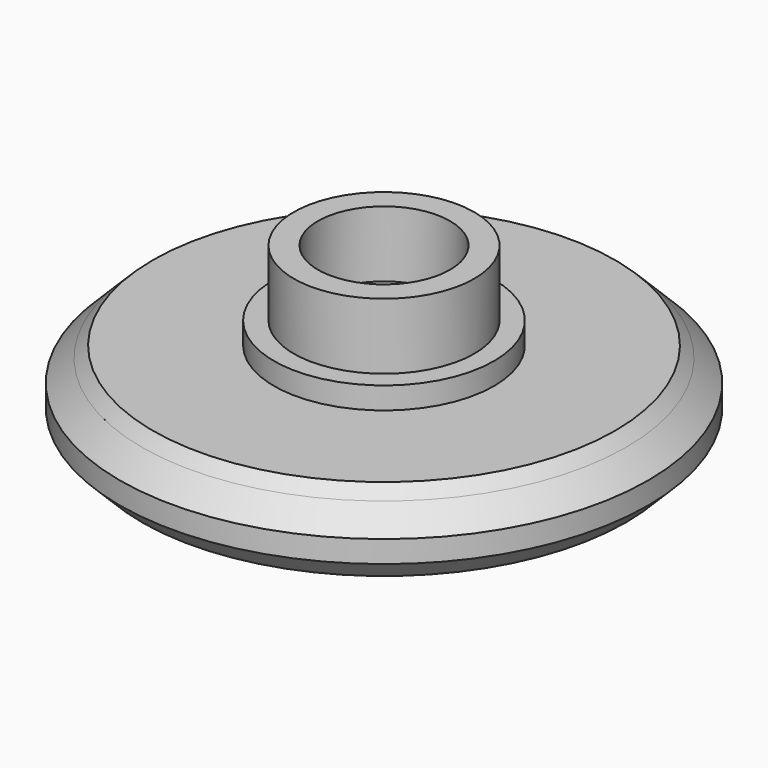
from build123d import *

# Parameters (mm, degrees)
F0_R     = 12
F0_R_2   = 11
F0_R_3   = 5
F0_R_4   = 4.1
F0_R_5   = 3
F1_DEPTH = 2
F2_DEPTH = 3.5
F3_SIZE  = 0.99999
F4_DEPTH = 4.5
F5_DEPTH = 7.5
F6_SIZE  = 1
F7_SIZE  = 0.5


# Not quite as in the source:
# - a fillet or chamfer is up to 0.001 mm smaller than in the source, because OpenCascade refuses the exact size


with BuildPart() as f1:
    # F0 (on Top) → F1 (new body)
    with BuildSketch(Plane.XY):
        Circle(F0_R)
        Circle(F0_R_2, mode=Mode.SUBTRACT)
        Circle(F0_R_2)
        Circle(F0_R_3, mode=Mode.SUBTRACT)
        Circle(F0_R_3)
        Circle(F0_R_4, mode=Mode.SUBTRACT)
        Circle(F0_R_4)
        Circle(F0_R_5, mode=Mode.SUBTRACT)
        Circle(F0_R_5)
    extrude(amount=F1_DEPTH)

    # F0 (on Top) → F2 (join)
    with BuildSketch(Plane.XY):
        Circle(F0_R_2)
        Circle(F0_R_3, mode=Mode.SUBTRACT)
        Circle(F0_R_3)
        Circle(F0_R_4, mode=Mode.SUBTRACT)
        Circle(F0_R_4)
        Circle(F0_R_5, mode=Mode.SUBTRACT)
        Circle(F0_R_5)
    extrude(amount=F2_DEPTH)

    # F3 (size 1 in the source; OpenCascade refuses exactly that, so slightly less here)
    f3_edges = [f1.edges().sort_by_distance(p)[0] for p in [
        (-11, 0, 2),
    ]]
    chamfer(f3_edges, length=F3_SIZE)

    # F0 (on Top) → F4 (join)
    with BuildSketch(Plane.XY):
        Circle(F0_R_3)
        Circle(F0_R_4, mode=Mode.SUBTRACT)
        Circle(F0_R_4)
        Circle(F0_R_5, mode=Mode.SUBTRACT)
        Circle(F0_R_5)
    extrude(amount=F4_DEPTH)

    # F0 (on Top) → F5 (join)
    with BuildSketch(Plane.XY):
        Circle(F0_R_4)
        Circle(F0_R_5, mode=Mode.SUBTRACT)
    extrude(amount=F5_DEPTH)

    # F6
    f6_edges = [f1.edges().sort_by_distance(p)[0] for p in [
        (-12, 0, 0),
    ]]
    chamfer(f6_edges, length=F6_SIZE)

    # F7
    f7_edges = [f1.edges().sort_by_distance(p)[0] for p in [
        (-11, 0, 3.5),
    ]]
    chamfer(f7_edges, length=F7_SIZE)


solid = f1.part
